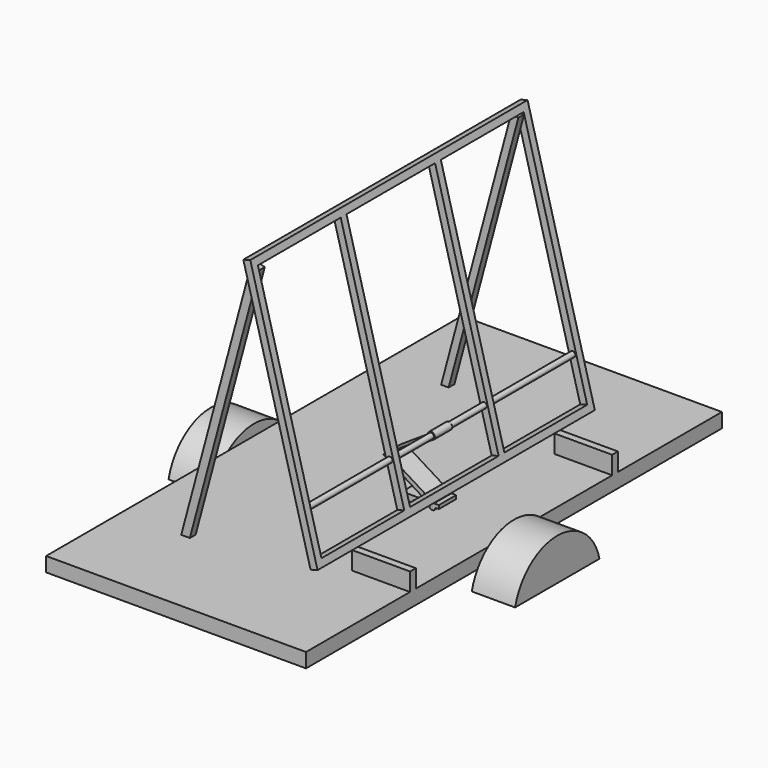
from build123d import *

# Parameters (mm, degrees)
F0_W      = 1828.8
F0_H      = 3657.6
F1_DEPTH  = 101.6
F3_DEPTH  = 304.8
F5_W      = 406.4
F5_H      = 50.8
F6_DEPTH  = 127
F8_DEPTH  = 2133.6
F9_DEPTH  = 304.8
F10_W     = 728.1164
F10_H     = 1727.2
F10_W_2   = 778.9672
F11_DEPTH = 1757.5817005799
F12_R     = 19.05
F13_DEPTH = 2438.4
F15_R     = 19.177
F16_DEPTH = 76.2
F18_DEPTH = 50.8
F20_DEPTH = 50.8


# Not quite as in the source:
# - a pattern or mirror of a feature is missing from the dataset's text; its kind, count and spacing are read off the source's solid


with BuildPart() as f1:
    # F0 (on Top) → F1 (new body)
    with BuildSketch(Plane.XY):
        with Locations((914.4, 1828.8)):
            Rectangle(F0_W, F0_H)
    extrude(amount=-F1_DEPTH)

    # F2 (on Right) → F3 (join)
    with BuildSketch(Plane.YZ):
        with BuildLine():
            Line((1457.8725633512, -217.7722070765), (2199.7274366488, -217.7722070765))
            ThreePointArc((2199.7274366488, -217.7722070765), (1828.8, 76.2), (1457.8725633512, -217.7722070765))
        make_face()
    f3 = extrude(amount=-F3_DEPTH)

    # F3_copies: F3 across plane
    add(f3.mirror(Plane(origin=(914.4, 0, 0), x_dir=(0, 0, 1), z_dir=(1, 0, 0))))

    # F5 (on face) → F6 (join)
    with BuildSketch(Plane.XY):
        with Locations((1625.6, 939.8)):
            Rectangle(F5_W, F5_H)
        with Locations((1625.6, 2717.8)):
            Rectangle(F5_W, F5_H)
    extrude(amount=F6_DEPTH)


with BuildPart() as f8:
    # F7 (on face) → F8 (new body)
    with BuildSketch(Plane.XZ.offset(-914.4)):
        Polygon((1373.3309680245, 113.8519925088), (1422.4, 127), (949.0717303165, 1893.4851511174), (900.002698341, 1880.3371436262), align=None)
    extrude(amount=-F8_DEPTH)

    # F7 (on face) → F9 (join)
    with BuildSketch(Plane.XZ.offset(-914.4)):
        Polygon((1373.3309680245, 113.8519925088), (1422.4, 127), (949.0717303165, 1893.4851511174), (900.002698341, 1880.3371436262), align=None)
    extrude(amount=F9_DEPTH)

    # F10 (on face) → F11 (cut, through all)
    with BuildSketch(Plane(origin=(1358.8672671715, 0, 364.1073868597), x_dir=(0, 1, 0), z_dir=(0.9659258263, 0, 0.2588190451))):
        with Locations((1024.4582, 668.9283701849)):
            Rectangle(F10_W, F10_H)
        with Locations((2633.1418, 668.9283701849)):
            Rectangle(F10_W, F10_H)
        with Locations((1828.8, 668.9283701849)):
            Rectangle(F10_W_2, F10_H)
    extrude(amount=-F11_DEPTH, mode=Mode.SUBTRACT)

    # F12 (on face) → F13 (join)
    with BuildSketch(Plane.XZ.offset(-609.6)):
        with Locations((1307.6271616768, 457.2)):
            Circle(F12_R)
    extrude(amount=-F13_DEPTH)


with BuildPart() as f16:
    # F15 (on offset) → F16 (new body, symmetric)
    with BuildSketch(Plane.XZ.offset(-1828.8)):
        with BuildLine():
            Line((1018.1603394521, 237.7031047405), (1314.0505465733, 432.6256205272))
            ThreePointArc((1314.0505465733, 432.6256205272), (1315.7904914246, 481.2524436894), (1287.5728110962, 441.6120872856))
            Line((1287.5728110962, 441.6120872856), (969.2683602777, 231.9238216842))
            Line((969.2683602777, 231.9238216842), (1237.3403362105, 65.2844932284))
            Line((1237.3403362105, 65.2844932284), (1281.3311466944, 45.2877443791))
            Line((1281.3311466944, 45.2877443791), (1103.3545091502, 45.2877443791))
            Line((1103.3545091502, 45.2877443791), (1103.3545091502, 20.3464620363))
            Line((1103.3545091502, 20.3464620363), (1138.9464007844, 20.3464620363))
            ThreePointArc((1138.9464007844, 20.3464620363), (1160.242493426, -0.9496306053), (1181.5385860676, 20.3464620363))
            Line((1181.5385860676, 20.3464620363), (1294.2654747231, 20.3464620363))
            ThreePointArc((1294.2654747231, 20.3464620363), (1315.4874399058, -0.8755031465), (1336.7094050886, 20.3464620363))
            Line((1336.7094050886, 20.3464620363), (1361.0237195842, 20.3464620363))
            Line((1361.0237195842, 20.3464620363), (1361.0237195842, 45.2877443791))
            Line((1361.0237195842, 45.2877443791), (1327.6981078161, 45.2877443791))
            Line((1327.6981078161, 45.2877443791), (1018.1603394521, 237.7031047405))
        make_face()
        with Locations((1307.6271616768, 457.2)):
            Circle(F15_R, mode=Mode.SUBTRACT)
    extrude(amount=F16_DEPTH, both=True)


with BuildPart() as f18:
    # F17 (on face) → F18 (new body)
    with BuildSketch(Plane(origin=(0, 660.4, 0), x_dir=(-1, 0, 0), z_dir=(0, 1, 0))):
        Polygon((-422.4638941905, 0), (-913.1507058322, 1831.2681116508), (-969.8107434721, 1816.086100322), (-483.1919395054, 0), align=None)
    extrude(amount=F18_DEPTH)


with BuildPart() as f20:
    # F19 (on face) → F20 (new body)
    with BuildSketch(Plane.XZ.offset(-2997.2)):
        Polygon((965.7427357971, 1831.2681116508), (913.1507058322, 1831.2681116508), (422.4638941905, 0), (475.0559241553, 0), align=None)
    extrude(amount=F20_DEPTH)


solid = Compound([f1.part, f8.part, f16.part, f18.part, f20.part])
